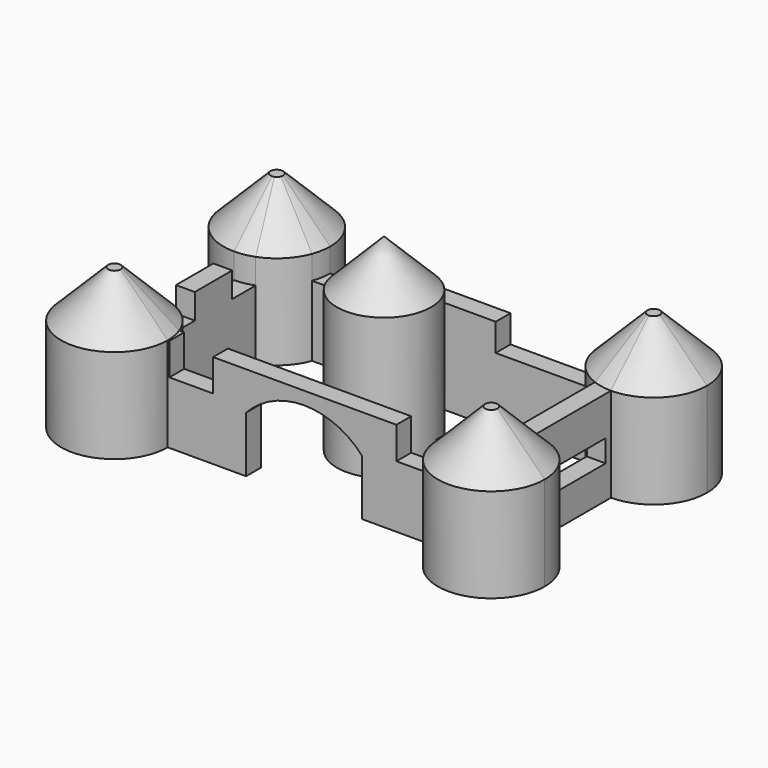
from build123d import *

# Parameters (mm, degrees)
F1_DEPTH   = 25.4
F2_DEPTH   = 38.1
F0_R       = 12.7
F3_DEPTH   = 50.8
F5_DEPTH   = 25.4
F4_W       = 11.7844194174
F4_H       = 8.6537211478
F4_W_2     = 10.750696063
F6_DEPTH   = 25.4
F7_W       = 1.4892533321
F7_H       = 6.7930224627
F7_W_2     = 6.9872582432
F7_W_3     = 6.3670262795
F7_W_4     = 2.1094843645
F8_DEPTH   = 25.4
F9_W       = 23.5688369721
F9_H       = 5.9955809265
F10_DEPTH  = 25.4
F11_W      = 1.8297875876
F11_H      = 7.4132553577
F11_W_2    = 24.2199800333
F11_W_3    = 22.1525379812
F11_H_2    = 6.3795357287
F11_W_4    = 3.6904881353
F12_DEPTH  = 25.4
F13_SIZE   = 12.7
F14_SIZE   = 12.7
F14_2_SIZE = 12.7
F14_3_SIZE = 12.7
F14_4_SIZE = 12.7


with BuildPart() as f1:
    # F0 (on Top) → F1 (new body)
    with BuildSketch(Plane.XY):
        with BuildLine():
            ThreePointArc((37.3095583182, 22.3796591884), (36.6425597983, 24.8327488181), (36.417887116, 27.364952985))
            Line((36.417887116, 27.364952985), (-36.417887116, 27.364952985))
            ThreePointArc((-36.417887116, 27.364952985), (-36.6425597983, 24.8327488181), (-37.3095583182, 22.3796591884))
            Line((-37.3095583182, 22.3796591884), (37.3095583182, 22.3796591884))
        make_face()
    extrude(amount=F1_DEPTH)

    # F11 (on face) → F12 (cut)
    with BuildSketch(Plane(origin=(0, 27.364952985, 0), x_dir=(-1, 0, 0), z_dir=(0, 1, 0))):
        with Locations((-37.3327809098, 21.6933723211)):
            Rectangle(F11_W, F11_H)
        with Locations((-24.3078970994, 21.6933723211)):
            Rectangle(F11_W_2, F11_H)
        with Locations((25.3416181254, 22.2102321357)):
            Rectangle(F11_W_3, F11_H_2)
        with Locations((38.2631311837, 22.2102321357)):
            Rectangle(F11_W_4, F11_H_2)
    extrude(amount=-F12_DEPTH, mode=Mode.SUBTRACT)


with BuildPart() as f1b:
    # F0 (on Top) → F1, piece 2 (new body)
    with BuildSketch(Plane.XY):
        with BuildLine():
            ThreePointArc((-45.72, 13.909888102), (-48.2180521889, 13.2165001894), (-50.8, 12.982840101))
            Line((-50.8, 12.982840101), (-50.8, -12.982840101))
            ThreePointArc((-50.8, -12.982840101), (-48.2180521889, -13.2165001894), (-45.72, -13.909888102))
            Line((-45.72, -13.909888102), (-45.72, 13.909888102))
        make_face()
    extrude(amount=F1_DEPTH)

    # F7 (on face) → F8 (cut)
    with BuildSketch(Plane(origin=(-50.8, 0, 0), x_dir=(0, -1, 0), z_dir=(-1, 0, 0))):
        with Locations((-13.7274667671, 22.0034887686)):
            Rectangle(F7_W, F7_H)
        with Locations((-9.4892109794, 22.0034887686)):
            Rectangle(F7_W_2, F7_H)
        with Locations((9.7993269613, 22.0034887686)):
            Rectangle(F7_W_3, F7_H)
        with Locations((14.0375822833, 22.0034887686)):
            Rectangle(F7_W_4, F7_H)
    extrude(amount=-F8_DEPTH, mode=Mode.SUBTRACT)


with BuildPart() as f1c:
    # F0 (on Top) → F1, piece 3 (new body)
    with BuildSketch(Plane.XY):
        with BuildLine():
            Line((50.8, -12.982840101), (50.8, 12.982840101))
            ThreePointArc((50.8, 12.982840101), (48.2180521889, 13.2165001894), (45.72, 13.909888102))
            Line((45.72, 13.909888102), (45.72, -13.909888102))
            ThreePointArc((45.72, -13.909888102), (48.2180521889, -13.2165001894), (50.8, -12.982840101))
        make_face()
    extrude(amount=F1_DEPTH)

    # F9 (on face) → F10 (cut)
    with BuildSketch(Plane.YZ.offset(50.8)):
        with Locations((-0.620232895, 11.8877906352)):
            Rectangle(F9_W, F9_H)
    extrude(amount=-F10_DEPTH, mode=Mode.SUBTRACT)


with BuildPart() as f1d:
    # F0 (on Top) → F1, piece 4 (new body)
    with BuildSketch(Plane.XY):
        with BuildLine():
            ThreePointArc((-37.3095583182, -22.3796591884), (-36.6425597983, -24.8327488181), (-36.417887116, -27.364952985))
            Line((-36.417887116, -27.364952985), (36.417887116, -27.364952985))
            ThreePointArc((36.417887116, -27.364952985), (36.6425597983, -24.8327488181), (37.3095583182, -22.3796591884))
            Line((37.3095583182, -22.3796591884), (-37.3095583182, -22.3796591884))
        make_face()
    extrude(amount=F1_DEPTH)

    # F4 (on face) → F5 (cut)
    with BuildSketch(Plane.XZ.offset(27.364952985)):
        with BuildLine():
            Line((-15.2990696952, 15.0923253968), (-15.2990696952, 0))
            Line((-15.2990696952, 0), (15.9193035215, 0))
            Line((15.9193035215, 0), (15.9193035215, 15.0923253968))
            ThreePointArc((15.9193035215, 15.0923253968), (0.3101169132, 21.9341960604), (-15.2990696952, 15.0923253968))
        make_face()
    extrude(amount=-F5_DEPTH, mode=Mode.SUBTRACT)

    # F4 (on face) → F6 (cut)
    with BuildSketch(Plane.XZ.offset(27.364952985)):
        with Locations((-30.0812795758, 21.0731394261)):
            Rectangle(F4_W, F4_H)
        with Locations((30.598141253, 21.0731394261)):
            Rectangle(F4_W_2, F4_H)
    extrude(amount=-F6_DEPTH, mode=Mode.SUBTRACT)


with BuildPart() as f2:
    # F0 (on Top) → F2 (new body)
    with BuildSketch(Plane.XY):
        with BuildLine():
            ThreePointArc((-37.3095583182, 22.3796591884), (-36.6425597983, 24.8327488181), (-36.417887116, 27.364952985))
            ThreePointArc((-36.417887116, 27.364952985), (-60.969689548, 37.534642533), (-50.8, 12.982840101))
            ThreePointArc((-50.8, 12.982840101), (-48.2180521889, 13.2165001894), (-45.72, 13.909888102))
            ThreePointArc((-45.72, 13.909888102), (-40.5946297653, 17.2310697521), (-37.3095583182, 22.3796591884))
        make_face()
    extrude(amount=F2_DEPTH)

    # F14
    f14_edges = [f2.edges().sort_by_distance(p)[0] for p in [
        (-50.8, 41.747066, 38.1),
    ]]
    chamfer(f14_edges, length=F14_SIZE)


with BuildPart() as f2b:
    # F0 (on Top) → F2, piece 2 (new body)
    with BuildSketch(Plane.XY):
        with BuildLine():
            ThreePointArc((65.182112884, 27.364952985), (50.8, 41.747065869), (36.417887116, 27.364952985))
            ThreePointArc((36.417887116, 27.364952985), (36.6425597983, 24.8327488181), (37.3095583182, 22.3796591884))
            ThreePointArc((37.3095583182, 22.3796591884), (40.5946297653, 17.2310697521), (45.72, 13.909888102))
            ThreePointArc((45.72, 13.909888102), (48.2180521889, 13.2165001894), (50.8, 12.982840101))
            ThreePointArc((50.8, 12.982840101), (60.969689548, 17.195263437), (65.182112884, 27.364952985))
        make_face()
    extrude(amount=F2_DEPTH)

    # F14#2
    f14_2_edges = [f2b.edges().sort_by_distance(p)[0] for p in [
        (65.182113, 27.364953, 38.1),
    ]]
    chamfer(f14_2_edges, length=F14_2_SIZE)


with BuildPart() as f2c:
    # F0 (on Top) → F2, piece 3 (new body)
    with BuildSketch(Plane.XY):
        with BuildLine():
            ThreePointArc((65.182112884, -27.364952985), (60.969689548, -17.195263437), (50.8, -12.982840101))
            ThreePointArc((50.8, -12.982840101), (48.2180521889, -13.2165001894), (45.72, -13.909888102))
            ThreePointArc((45.72, -13.909888102), (40.5946297653, -17.2310697521), (37.3095583182, -22.3796591884))
            ThreePointArc((37.3095583182, -22.3796591884), (36.6425597983, -24.8327488181), (36.417887116, -27.364952985))
            ThreePointArc((36.417887116, -27.364952985), (50.8, -41.747065869), (65.182112884, -27.364952985))
        make_face()
    extrude(amount=F2_DEPTH)

    # F14#3
    f14_3_edges = [f2c.edges().sort_by_distance(p)[0] for p in [
        (36.417887, -27.364953, 38.1),
    ]]
    chamfer(f14_3_edges, length=F14_3_SIZE)


with BuildPart() as f2d:
    # F0 (on Top) → F2, piece 4 (new body)
    with BuildSketch(Plane.XY):
        with BuildLine():
            ThreePointArc((-45.72, -13.909888102), (-48.2180521889, -13.2165001894), (-50.8, -12.982840101))
            ThreePointArc((-50.8, -12.982840101), (-60.969689548, -37.534642533), (-36.417887116, -27.364952985))
            ThreePointArc((-36.417887116, -27.364952985), (-36.6425597983, -24.8327488181), (-37.3095583182, -22.3796591884))
            ThreePointArc((-37.3095583182, -22.3796591884), (-40.5946297653, -17.2310697521), (-45.72, -13.909888102))
        make_face()
    extrude(amount=F2_DEPTH)

    # F14#4
    f14_4_edges = [f2d.edges().sort_by_distance(p)[0] for p in [
        (-65.182113, -27.364953, 38.1),
    ]]
    chamfer(f14_4_edges, length=F14_4_SIZE)


with BuildPart() as f3:
    # F0 (on Top) → F3 (new body)
    with BuildSketch(Plane.XY):
        Circle(F0_R)
    extrude(amount=F3_DEPTH)

    # F13
    f13_edges = [f3.edges().sort_by_distance(p)[0] for p in [
        (-12.7, 0, 50.8),
    ]]
    chamfer(f13_edges, length=F13_SIZE)


solid = Compound([f1.part, f1b.part, f1c.part, f1d.part, f2.part, f2b.part, f2c.part, f2d.part, f3.part])
